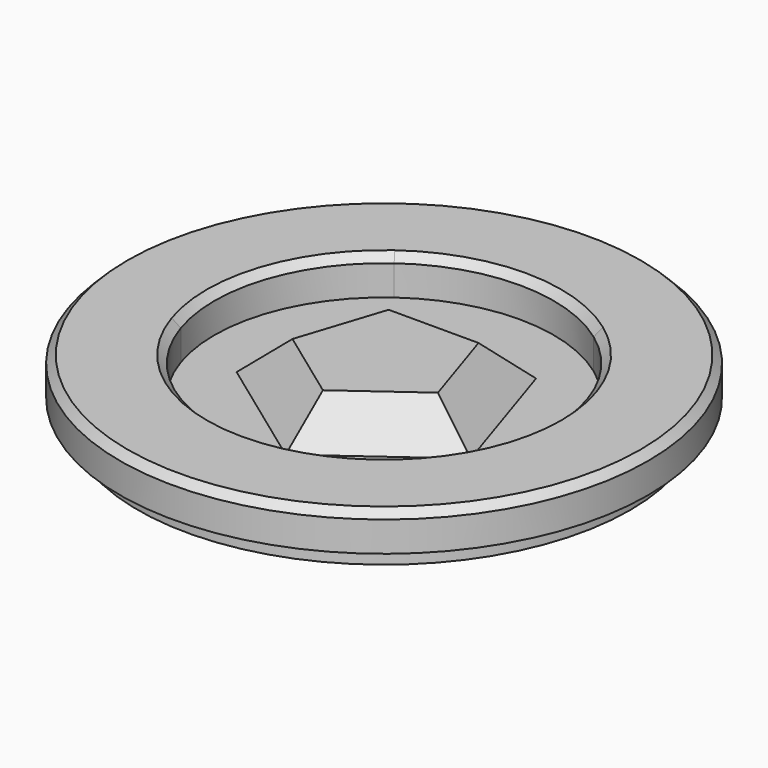
from build123d import *

# Parameters (mm, degrees)
F0_R        = 17.78
F1_DEPTH    = 2.54
F2_SIZE     = 0.508
F3_T1_DEPTH = 39.5650700251
F3_T3_DEPTH = 39.5650700251
F3_T5_DEPTH = 39.5650700251
F3_T7_DEPTH = 39.5650700251
F3_T9_DEPTH = 39.5650700251
F4_R        = 16.580892073
F5_DEPTH    = 1.27


# Not quite as in the source:
# - a fillet or chamfer that OpenCascade refuses, or shapes differently, is made with other operations: its cross-section is extruded or revolved along the edge and cut away or added


with BuildPart() as f1:
    # F0 (on Top) → F1 (new body)
    with BuildSketch(Plane.XY):
        Circle(F0_R)
        with BuildLine():
            ThreePointArc((6.7183854337, 9.2470642457), (10.1842045715, 5.189111412), (11.43, 0))
            ThreePointArc((11.43, 0), (11.289277733, -1.7880459354), (10.8705759813, -3.5320642457))
            ThreePointArc((10.8705759813, -3.5320642457), (6.7183854337, -9.2470642457), (0, -11.43))
            ThreePointArc((0, -11.43), (-6.7183854337, -9.2470642457), (-10.8705759813, -3.5320642457))
            ThreePointArc((-10.8705759813, -3.5320642457), (-10.8705759813, 3.5320642457), (-6.7183854337, 9.2470642457))
            ThreePointArc((-6.7183854337, 9.2470642457), (0, 11.43), (6.7183854337, 9.2470642457))
        make_face(mode=Mode.SUBTRACT)
    extrude(amount=F1_DEPTH)

    # F2
    f2_edges = [f1.edges().sort_by_distance(p)[0] for p in [
        (-17.78, 0, 2.54),
        (0, 11.43, 2.54),
    ]]
    chamfer(f2_edges, length=F2_SIZE)


with BuildPart() as f1b:
    # F0 (on Top) → F1, piece 2 (new body)
    with BuildSketch(Plane.XY):
        Polygon((10.8705759813, -3.5320642457), (6.7183854337, 9.2470642457), (-6.7183854337, 9.2470642457), (-10.8705759813, -3.5320642457), (0, -11.43), align=None)
    extrude(amount=F1_DEPTH)

    # F3: chamfer of 5.08 on 5 edges, made by hand

    # F3_s2 → F3_t1 (cut)
    with BuildSketch(Plane(origin=(-16.004407017, 11.6278823333, 0), x_dir=(0, 0, 1), z_dir=(0.8090169944, -0.5877852523, 0))):
        Polygon((-2.54, 9.2470642457), (2.54, 4.1670642457), (2.54, 9.2470642457), align=None)
    extrude(amount=F3_T1_DEPTH, mode=Mode.SUBTRACT)

    # F3_s4 → F3_t3 (cut)
    with BuildSketch(Plane(origin=(-16.004407017, -11.6278823333, 0), x_dir=(0, 0, 1), z_dir=(0.8090169944, 0.5877852523, 0))):
        Polygon((-2.54, 9.2470642457), (2.54, 4.1670642457), (2.54, 9.2470642457), align=None)
    extrude(amount=F3_T3_DEPTH, mode=Mode.SUBTRACT)

    # F3_s6 → F3_t5 (cut)
    with BuildSketch(Plane(origin=(6.1131395107, -18.8143088325, 0), x_dir=(0, 0, 1), z_dir=(-0.3090169944, 0.9510565163, 0))):
        Polygon((-2.54, 9.2470642457), (2.54, 4.1670642457), (2.54, 9.2470642457), align=None)
    extrude(amount=F3_T5_DEPTH, mode=Mode.SUBTRACT)

    # F3_s8 → F3_t7 (cut)
    with BuildSketch(Plane.YZ.offset(-19.7825350126)):
        Polygon((9.2470642457, -2.54), (4.1670642457, 2.54), (9.2470642457, 2.54), align=None)
    extrude(amount=F3_T7_DEPTH, mode=Mode.SUBTRACT)

    # F3_s10 → F3_t9 (cut)
    with BuildSketch(Plane(origin=(6.1131395107, 18.8143088325, 0), x_dir=(0, 0, 1), z_dir=(-0.3090169944, -0.9510565163, 0))):
        Polygon((-2.54, 9.2470642457), (2.54, 4.1670642457), (2.54, 9.2470642457), align=None)
    extrude(amount=F3_T9_DEPTH, mode=Mode.SUBTRACT)


with BuildPart() as f5:
    # F4 (on Top) → F5 (new body)
    with BuildSketch(Plane.XY):
        Circle(F4_R)
    extrude(amount=-F5_DEPTH)


solid = Compound([f1.part, f1b.part, f5.part])
